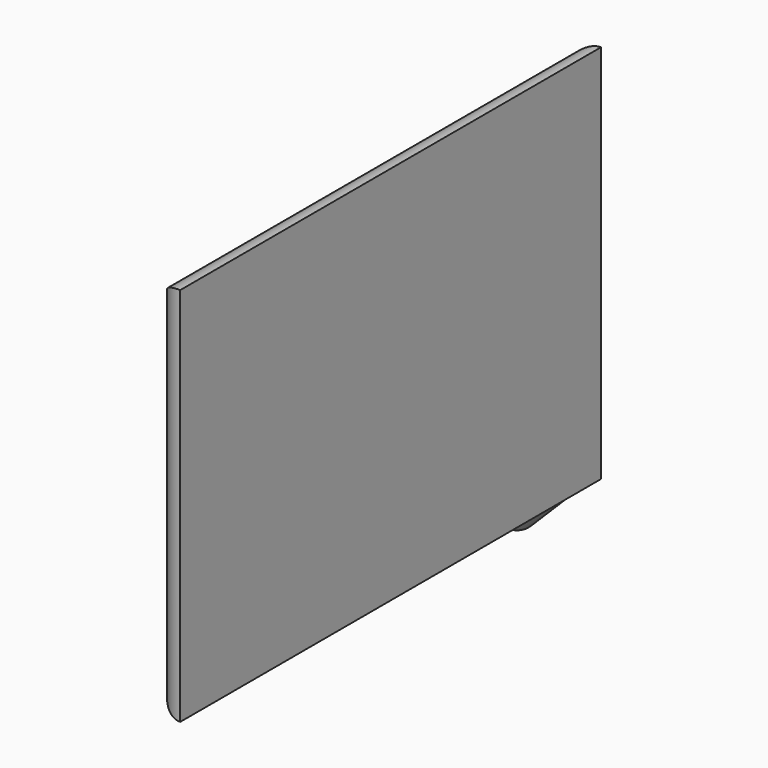
from build123d import *

# Parameters (mm, degrees)
F0_W     = 97.2719080746
F0_H     = 70.3038610518
F1_DEPTH = 5.08
F2_R     = 5.07999
F4_R     = 5.5791141454
F5_DEPTH = 12


# Not quite as in the source:
# - a fillet or chamfer is up to 0.001 mm smaller than in the source, because OpenCascade refuses the exact size


with BuildPart() as f1:
    # F0 (on Right) → F1 (new body)
    with BuildSketch(Plane.YZ):
        with Locations((6.223058328, -2.6357788593)):
            Rectangle(F0_W, F0_H)
    extrude(amount=-F1_DEPTH)

    # F2 (radius 5.08 in the source; OpenCascade refuses exactly that, so slightly less here)
    f2_edges = [f1.edges().sort_by_distance(p)[0] for p in [
        (-5.08, 6.223058, 32.516152),
        (-5.08, -42.412896, -2.635779),
        (-5.08, 6.223058, -37.787709),
        (-5.08, 54.859012, -2.635779),
    ]]
    fillet(f2_edges, radius=F2_R)

    # F4 (on line) → F5 (join)
    with BuildSketch(Plane(origin=(-18.8938546926, 0, -18.8938546926), x_dir=(0.7071067812, 0, -0.7071067812), z_dir=(0.7071067812, 0, 0.7071067812))):
        with Locations((20.8907071501, 48.9649102092)):
            Circle(F4_R)
    extrude(amount=-F5_DEPTH)

    # F5_face (on face) → F6 (join, up to the last surface of F1)
    with BuildSketch(Plane(origin=(-6.0444772331, 49.5744646738, -31.743232152), x_dir=(0.7071067812, 0, -0.7071067812), z_dir=(0.7071067812, 0, 0.7071067812))):
        with BuildLine():
            add(Edge.make_bspline(
                [(4.8341488182, 4.5530437353), (1.3639767837, 3.0711160289), (1.3639767837, 0.2045576915)],
                knots=[5.255697667, 5.255697667, 5.255697667, 6.2831853072, 6.2831853072, 6.2831853072], degree=2, weights=[1, 0.8709107479, 1]))
            ThreePointArc((4.8341488182, 4.5530437353), (-2.582040706, 1.1300096876), (1.3639767837, -6.021631741))
            Line((1.3639767837, -6.021631741), (1.3639767837, 0.2045576915))
        make_face()
    extrude(until=Until.LAST)


solid = f1.part
